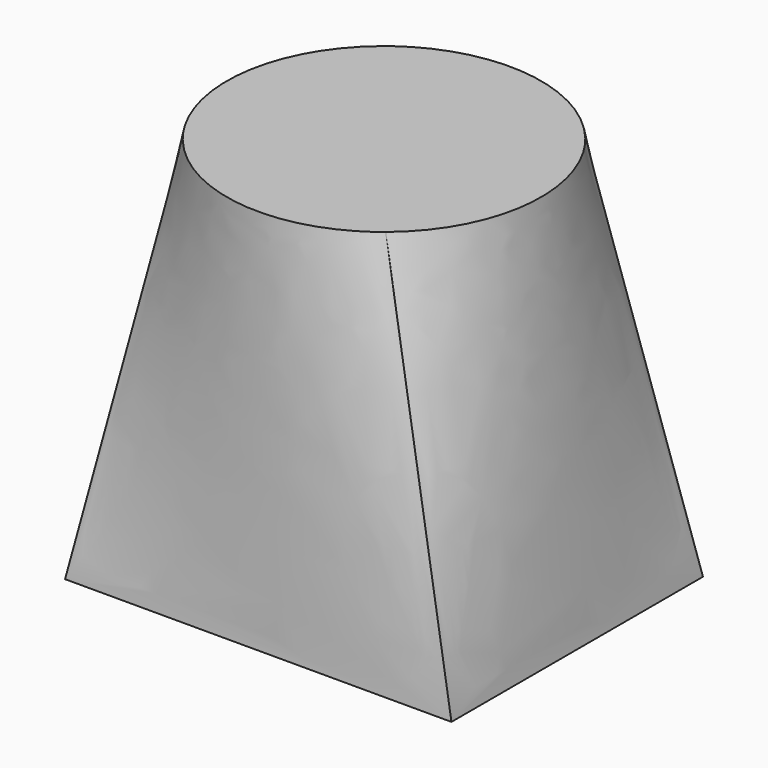
from build123d import *

# Parameters (mm, degrees)
F0_W = 50.8
F0_H = 41.3327284643
F4_T = 2.286


# Not quite as in the source:
# - the arcs of a loft's sections are written as splines that run evenly, so that the points pair up as in the source's solid
# - a shell that OpenCascade refuses in one call is made with other operations: the cavity is built on its own and cut out


with BuildPart() as f3:
    # F0 (on Top) → F3 section 0
    with BuildSketch(Plane.XY):
        Rectangle(F0_W, F0_H)
    # F2 (on offset) → F3 section 1
    with BuildSketch(Plane.XY.offset(50.8)):
        with BuildLine():
            add(Edge.make_bspline(
                [(16.0305352967, 13.0430268219), (15.1768711874, 14.0922229036), (14.2198939474, 15.0573165448), (12.135995559, 16.7823054792), (11.0091259391, 17.5421581187), (8.6287404272, 18.8274534668), (7.3752833949, 19.3528643939), (4.7898876398, 20.1490729763), (3.458012846, 20.4198509437), (0.7669621567, 20.696374911), (-0.5921471973, 20.7021140733), (-3.2854372521, 20.4483267645), (-4.6195513559, 20.1888065689), (-7.2115791497, 19.414460888), (-8.4694287466, 18.8996545501), (-10.8605841049, 17.6345081674), (-11.9938307403, 16.8841994059), (-13.0430268219, 16.0305352967)],
                knots=[0, 0, 0, 0, 0.125, 0.125, 0.25, 0.25, 0.375, 0.375, 0.5, 0.5, 0.625, 0.625, 0.75, 0.75, 0.875, 0.875, 1, 1, 1, 1], degree=3))
            add(Edge.make_bspline(
                [(-13.0430268219, 16.0305352967), (-14.0922229036, 15.1768711874), (-15.0573165448, 14.2198939474), (-16.7823054792, 12.135995559), (-17.5421581187, 11.0091259391), (-18.8274534668, 8.6287404272), (-19.3528643939, 7.3752833949), (-20.1490729763, 4.7898876398), (-20.4198509437, 3.458012846), (-20.696374911, 0.7669621567), (-20.7021140733, -0.5921471973), (-20.4483267645, -3.2854372521), (-20.1888065689, -4.6195513559), (-19.414460888, -7.2115791497), (-18.8996545501, -8.4694287466), (-17.6345081674, -10.8605841049), (-16.8841994059, -11.9938307403), (-16.0305352967, -13.0430268219)],
                knots=[0, 0, 0, 0, 0.125, 0.125, 0.25, 0.25, 0.375, 0.375, 0.5, 0.5, 0.625, 0.625, 0.75, 0.75, 0.875, 0.875, 1, 1, 1, 1], degree=3))
            add(Edge.make_bspline(
                [(-16.0305352967, -13.0430268219), (-15.1768711874, -14.0922229036), (-14.2198939474, -15.0573165448), (-12.135995559, -16.7823054792), (-11.0091259391, -17.5421581187), (-8.6287404272, -18.8274534668), (-7.3752833949, -19.3528643939), (-4.7898876398, -20.1490729763), (-3.458012846, -20.4198509437), (-0.7669621567, -20.696374911), (0.5921471973, -20.7021140733), (3.2854372521, -20.4483267645), (4.6195513559, -20.1888065689), (7.2115791497, -19.414460888), (8.4694287466, -18.8996545501), (10.8605841049, -17.6345081674), (11.9938307403, -16.8841994059), (13.0430268219, -16.0305352967)],
                knots=[0, 0, 0, 0, 0.125, 0.125, 0.25, 0.25, 0.375, 0.375, 0.5, 0.5, 0.625, 0.625, 0.75, 0.75, 0.875, 0.875, 1, 1, 1, 1], degree=3))
            add(Edge.make_bspline(
                [(13.0430268219, -16.0305352967), (14.0922229036, -15.1768711874), (15.0573165448, -14.2198939474), (16.7823054792, -12.135995559), (17.5421581187, -11.0091259391), (18.8274534668, -8.6287404272), (19.3528643939, -7.3752833949), (20.1490729763, -4.7898876398), (20.4198509437, -3.458012846), (20.696374911, -0.7669621567), (20.7021140733, 0.5921471973), (20.4483267645, 3.2854372521), (20.1888065689, 4.6195513559), (19.414460888, 7.2115791497), (18.8996545501, 8.4694287466), (17.6345081674, 10.8605841049), (16.8841994059, 11.9938307403), (16.0305352967, 13.0430268219)],
                knots=[0, 0, 0, 0, 0.125, 0.125, 0.25, 0.25, 0.375, 0.375, 0.5, 0.5, 0.625, 0.625, 0.75, 0.75, 0.875, 0.875, 1, 1, 1, 1], degree=3))
        make_face()
    loft(ruled=True)

    # F4: shell of thickness 2.286, made by hand


with BuildPart() as f4_core1:
    # F4_t2: copy of F3
    add(f3.part)

    # the walls: a layer under each face that stays
    f4_faces = [f4_core1.faces().sort_by_distance(p)[0] for p in [
        (22.9790564637, -1.0562437507, 25.4),
        (1.0562437507, 20.6122385797, 25.4),
        (-22.9790564637, 1.0562437507, 25.4),
        (-1.0562437507, -20.6122385797, 25.4),
        (0, 0, 50.8),
    ]]
    thicken(f4_faces, amount=-F4_T, mode=Mode.SUBTRACT)


with BuildPart() as f3_1:
    add(f3.part)

    # what is left inside the walls is the cavity
    f4_cavity = [f4_core1.part.solids().sort_by_distance(p)[0] for p in [
        (-0.625568, -18.323309, 16.343336),
    ]]
    add(f4_cavity, mode=Mode.SUBTRACT)


solid = f3_1.part
